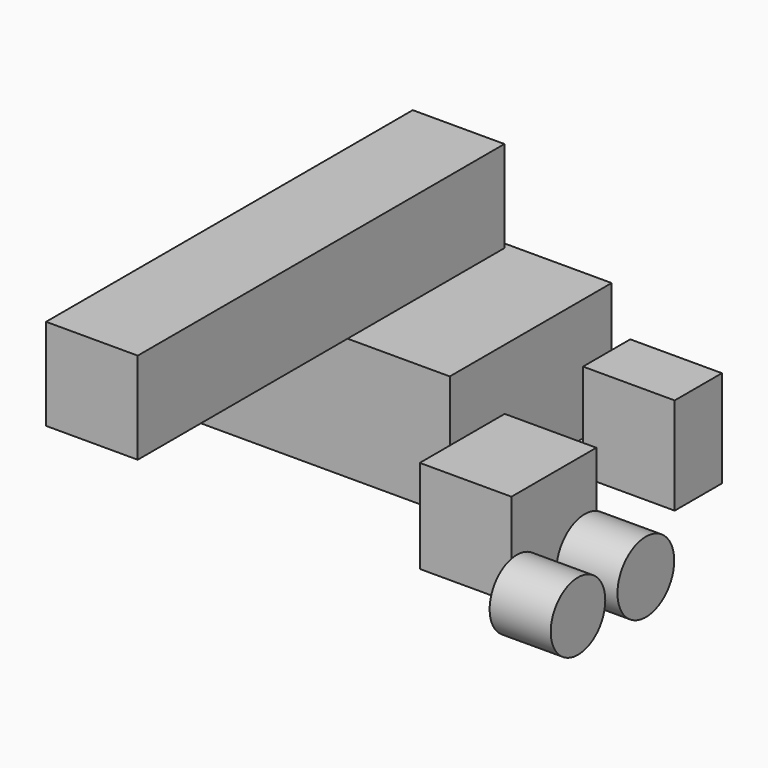
from build123d import *

# Parameters (mm, degrees)
F0_W     = 76.2
F0_H     = 76.2
F1_DEPTH = 381
F4_W     = 243.6232632026
F4_H     = 168.1647449732
F5_DEPTH = 101.6
F6_W     = 88.2032513618
F6_H     = 77.649012208
F6_W_2   = 49.0783378482
F6_H_2   = 80.6645080447
F7_DEPTH = 76.2
F8_R     = 28.3330362408
F8_R_2   = 29.4879309961
F9_DEPTH = 50.8


# Not quite as in the source:
# - the program builds the solid bodies; features that only make, move or delete a surface that nothing else refers to are left out


with BuildPart() as f1:
    # F0 (on Front) → F1 (new body)
    with BuildSketch(Plane.XZ):
        with Locations((-5.1436224073, 48.1359618664)):
            Rectangle(F0_W, F0_H)
    extrude(amount=F1_DEPTH)

    # F4 (on face) → F5 (join)
    with BuildSketch(Plane(origin=(0, 0, 10.0359618664), x_dir=(1, 0, 0), z_dir=(0, 0, -1))):
        with Locations((-3.8859811611, 78.9063498378)):
            Rectangle(F4_W, F4_H)
    extrude(amount=F5_DEPTH)

    # F6 (on face) → F7 (join)
    with BuildSketch(Plane.YZ.offset(117.9256504402)):
        with Locations((-150.0591784716, -79.3707072735)):
            Rectangle(F6_W, F6_H)
        with Locations((0, -79.3707072735)):
            Rectangle(F6_W_2, F6_H_2)
    extrude(amount=F7_DEPTH)

    # F8 (on face) → F9 (join)
    with BuildSketch(Plane.YZ.offset(194.1256504402)):
        with Locations((-188.5067522526, -113.6719733477)):
            Circle(F8_R)
        with Locations((-118.0195510387, -113.6719733477)):
            Circle(F8_R_2)
    extrude(amount=F9_DEPTH)


solid = f1.part
